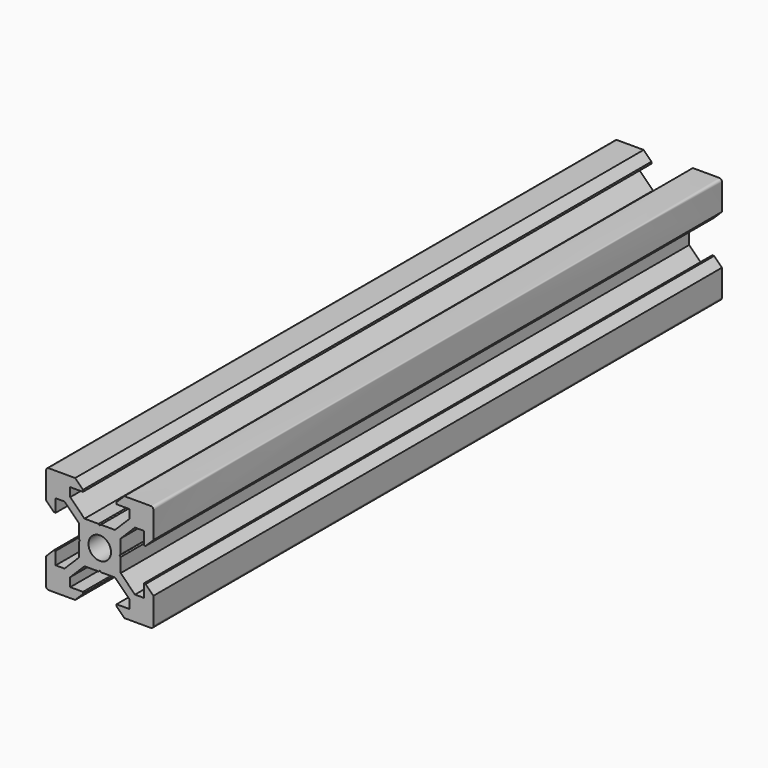
from build123d import *

# Parameters (mm, degrees)
F1_DEPTH = 132.4


# Not quite as in the source:
# - the dataset's text gives a spline's control points without its knots; the knots are read off the source's solid


with BuildPart() as f1:
    # F0 (on Front) → F1 (new body)
    with BuildSketch(Plane.XZ):
        with BuildLine():
            add(Edge.make_bspline(
                [(-8.545, 3.1250000004), (-8.43, 3.1250000004), (-8.315, 3.1250000004), (-8.2, 3.1250000004)],
                knots=[0, 0, 0, 0, 1, 1, 1, 1], degree=3))
            add(Edge.make_bspline(
                [(-8.2, 3.1250000004), (-8.2, 3.9166666671), (-8.2, 4.7083333338), (-8.2, 5.5000000004)],
                knots=[0, 0, 0, 0, 1, 1, 1, 1], degree=3))
            add(Edge.make_bspline(
                [(-8.1999999959, 5.5000000044), (-7.6535533893, 5.5000000044), (-7.1071067826, 5.5000000044), (-6.5606601759, 5.5000000044)],
                knots=[0, 0, 0, 0, 1, 1, 1, 1], degree=3))
            add(Edge.make_bspline(
                [(-6.5606601759, 5.5000000044), (-5.6737734493, 4.6131132778), (-4.7868867226, 3.7262265511), (-3.8999999959, 2.8393398244)],
                knots=[0, 0, 0, 0, 1, 1, 1, 1], degree=3))
            add(Edge.make_bspline(
                [(-3.8999999979, 2.8393398226), (-3.8999999979, 1.9628932159), (-3.8999999979, 1.0864466093), (-3.8999999979, 0.2100000026)],
                knots=[0, 0, 0, 0, 1, 1, 1, 1], degree=3))
            add(Edge.make_bspline(
                [(-3.9, 0.2100000008), (-3.83, 0.1400000008), (-3.76, 0.0700000008), (-3.69, 8e-10)],
                knots=[0, 0, 0, 0, 1, 1, 1, 1], degree=3))
            add(Edge.make_bspline(
                [(-3.9, -0.2099999992), (-3.83, -0.1399999992), (-3.76, -0.0699999992), (-3.69, 8e-10)],
                knots=[0, 0, 0, 0, 1, 1, 1, 1], degree=3))
            add(Edge.make_bspline(
                [(-3.8999999991, -2.839339821), (-3.8999999987, -1.9628932143), (-3.8999999984, -1.0864466077), (-3.899999998, -0.210000001)],
                knots=[0, 0, 0, 0, 1, 1, 1, 1], degree=3))
            add(Edge.make_bspline(
                [(-6.5606601782, -5.5000000017), (-5.6737734512, -4.6131132754), (-4.7868867241, -3.7262265491), (-3.8999999971, -2.8393398228)],
                knots=[0, 0, 0, 0, 1, 1, 1, 1], degree=3))
            add(Edge.make_bspline(
                [(-8.1999999982, -5.5000000011), (-7.6535533915, -5.5000000013), (-7.1071067849, -5.5000000015), (-6.5606601782, -5.5000000017)],
                knots=[0, 0, 0, 0, 1, 1, 1, 1], degree=3))
            add(Edge.make_bspline(
                [(-8.2000000012, -3.1249999971), (-8.2000000015, -3.9166666637), (-8.2000000019, -4.7083333304), (-8.2000000022, -5.4999999971)],
                knots=[0, 0, 0, 0, 1, 1, 1, 1], degree=3))
            add(Edge.make_bspline(
                [(-8.5450000012, -3.1249999969), (-8.4300000012, -3.124999997), (-8.3150000012, -3.124999997), (-8.2000000012, -3.1249999971)],
                knots=[0, 0, 0, 0, 1, 1, 1, 1], degree=3))
            add(Edge.make_bspline(
                [(-10.0000000018, -4.5799999963), (-9.5150000016, -4.0949999965), (-9.0300000014, -3.6099999967), (-8.5450000012, -3.1249999969)],
                knots=[0, 0, 0, 0, 1, 1, 1, 1], degree=3))
            add(Edge.make_bspline(
                [(-10.0000000038, -9.4999999963), (-10.0000000032, -7.8599999963), (-10.0000000025, -6.2199999963), (-10.0000000018, -4.5799999963)],
                knots=[0, 0, 0, 0, 1, 1, 1, 1], degree=3))
            add(Edge.make_bspline(
                [(-9.5000000039, -9.9999999965), (-9.5655199967, -9.9999999965), (-9.6293005688, -9.9873132519), (-9.6913417201, -9.9619397628), (-9.7513299005, -9.9374058943), (-9.8054004587, -9.9012771024), (-9.8535533945, -9.853553387), (-9.8995865416, -9.8079305653), (-9.9357153335, -9.7538600072), (-9.9619397702, -9.6913417126), (-9.9873132593, -9.6308520521), (-10.0000000039, -9.56707148), (-10.0000000038, -9.4999999963)],
                knots=[0, 0, 0, 0, 0.25, 0.25, 0.25, 0.5, 0.5, 0.5, 0.75, 0.75, 0.75, 1, 1, 1, 1], degree=3))
            add(Edge.make_bspline(
                [(-4.580000004, -9.9999999986), (-6.220000004, -9.9999999979), (-7.860000004, -9.9999999972), (-9.500000004, -9.9999999965)],
                knots=[0, 0, 0, 0, 1, 1, 1, 1], degree=3))
            Line((-4.580000004, -9.9999999986), (-3.1250000034, -8.5449999991))
            add(Edge.make_bspline(
                [(-3.1250000033, -8.1999999991), (-3.1250000033, -8.3149999991), (-3.1250000034, -8.4299999991), (-3.1250000034, -8.5449999991)],
                knots=[0, 0, 0, 0, 1, 1, 1, 1], degree=3))
            add(Edge.make_bspline(
                [(-5.5000000033, -8.1999999982), (-4.7083333366, -8.1999999985), (-3.91666667, -8.1999999988), (-3.1250000033, -8.1999999991)],
                knots=[0, 0, 0, 0, 1, 1, 1, 1], degree=3))
            add(Edge.make_bspline(
                [(-5.5000000066, -6.5606601742), (-5.5000000069, -7.1071067808), (-5.5000000071, -7.6535533875), (-5.5000000073, -8.1999999942)],
                knots=[0, 0, 0, 0, 1, 1, 1, 1], degree=3))
            add(Edge.make_bspline(
                [(-2.8393398255, -3.8999999953), (-3.7262265526, -4.7868867216), (-4.6131132796, -5.6737734479), (-5.5000000066, -6.5606601742)],
                knots=[0, 0, 0, 0, 1, 1, 1, 1], degree=3))
            add(Edge.make_bspline(
                [(-0.2100000015, -3.9000000003), (-1.0864466082, -3.9), (-1.9628932149, -3.8999999996), (-2.8393398215, -3.8999999993)],
                knots=[0, 0, 0, 0, 1, 1, 1, 1], degree=3))
            add(Edge.make_bspline(
                [(-1.5e-09, -3.6900000004), (-0.0700000015, -3.7600000004), (-0.1400000015, -3.8300000004), (-0.2100000015, -3.9000000003)],
                knots=[0, 0, 0, 0, 1, 1, 1, 1], degree=3))
            add(Edge.make_bspline(
                [(0.2099999985, -3.9000000005), (0.1399999985, -3.8300000005), (0.0699999985, -3.7600000005), (-1.5e-09, -3.6900000004)],
                knots=[0, 0, 0, 0, 1, 1, 1, 1], degree=3))
            add(Edge.make_bspline(
                [(2.8393398185, -3.9000000016), (1.9628932118, -3.9000000012), (1.0864466051, -3.9000000009), (0.2099999985, -3.9000000005)],
                knots=[0, 0, 0, 0, 1, 1, 1, 1], degree=3))
            add(Edge.make_bspline(
                [(5.4999999974, -6.5606601827), (4.6131132711, -5.6737734557), (3.7262265448, -4.7868867286), (2.8393398185, -3.9000000016)],
                knots=[0, 0, 0, 0, 1, 1, 1, 1], degree=3))
            add(Edge.make_bspline(
                [(5.4999999967, -8.2000000027), (5.4999999969, -7.653553396), (5.4999999971, -7.1071067894), (5.4999999974, -6.5606601827)],
                knots=[0, 0, 0, 0, 1, 1, 1, 1], degree=3))
            add(Edge.make_bspline(
                [(3.1249999967, -8.2000000017), (3.9166666634, -8.200000002), (4.70833333, -8.2000000024), (5.4999999967, -8.2000000027)],
                knots=[0, 0, 0, 0, 1, 1, 1, 1], degree=3))
            add(Edge.make_bspline(
                [(3.1249999966, -8.5450000017), (3.1249999966, -8.4300000017), (3.1249999967, -8.3150000017), (3.1249999967, -8.2000000017)],
                knots=[0, 0, 0, 0, 1, 1, 1, 1], degree=3))
            add(Edge.make_bspline(
                [(4.579999996, -10.0000000023), (4.0949999962, -9.5150000021), (3.6099999964, -9.0300000019), (3.1249999966, -8.5450000017)],
                knots=[0, 0, 0, 0, 1, 1, 1, 1], degree=3))
            add(Edge.make_bspline(
                [(9.499999996, -10.0000000043), (7.859999996, -10.0000000037), (6.219999996, -10.000000003), (4.579999996, -10.0000000023)],
                knots=[0, 0, 0, 0, 1, 1, 1, 1], degree=3))
            add(Edge.make_bspline(
                [(9.999999996, -9.5000000043), (9.999999996, -9.5655199971), (9.9873132515, -9.6293005692), (9.9619397623, -9.6913417205), (9.9374058938, -9.7513299009), (9.9012771019, -9.8054004591), (9.8535533866, -9.853553395), (9.8079305649, -9.899586542), (9.7538600068, -9.9357153339), (9.6913417122, -9.9619397706), (9.6308520517, -9.9873132598), (9.5670714797, -10.0000000043), (9.499999996, -10.0000000043)],
                knots=[0, 0, 0, 0, 0.25, 0.25, 0.25, 0.5, 0.5, 0.5, 0.75, 0.75, 0.75, 1, 1, 1, 1], degree=3))
            add(Edge.make_bspline(
                [(9.9999999981, -4.5800000043), (9.9999999974, -6.2200000043), (9.9999999967, -7.8600000043), (9.999999996, -9.5000000043)],
                knots=[0, 0, 0, 0, 1, 1, 1, 1], degree=3))
            add(Edge.make_bspline(
                [(8.5449999987, -3.1250000037), (9.0299999985, -3.6100000039), (9.5149999983, -4.0950000041), (9.9999999981, -4.5800000043)],
                knots=[0, 0, 0, 0, 1, 1, 1, 1], degree=3))
            add(Edge.make_bspline(
                [(8.1999999987, -3.1250000036), (8.3149999987, -3.1250000036), (8.4299999987, -3.1250000037), (8.5449999987, -3.1250000037)],
                knots=[0, 0, 0, 0, 1, 1, 1, 1], degree=3))
            add(Edge.make_bspline(
                [(8.1999999977, -5.5000000036), (8.199999998, -4.7083333369), (8.1999999983, -3.9166666703), (8.1999999987, -3.1250000036)],
                knots=[0, 0, 0, 0, 1, 1, 1, 1], degree=3))
            add(Edge.make_bspline(
                [(6.5606601777, -5.5000000019), (7.1071067843, -5.5000000022), (7.653553391, -5.5000000024), (8.1999999977, -5.5000000026)],
                knots=[0, 0, 0, 0, 1, 1, 1, 1], degree=3))
            add(Edge.make_bspline(
                [(3.8999999988, -2.8393398208), (4.7868867251, -3.7262265479), (5.6737734514, -4.6131132749), (6.5606601777, -5.5000000019)],
                knots=[0, 0, 0, 0, 1, 1, 1, 1], degree=3))
            add(Edge.make_bspline(
                [(3.8999999999, -0.2100000008), (3.8999999995, -1.0864466075), (3.8999999991, -1.9628932142), (3.8999999988, -2.8393398208)],
                knots=[0, 0, 0, 0, 1, 1, 1, 1], degree=3))
            add(Edge.make_bspline(
                [(3.69, -8e-10), (3.76, -0.0700000008), (3.8299999999, -0.1400000008), (3.8999999999, -0.2100000008)],
                knots=[0, 0, 0, 0, 1, 1, 1, 1], degree=3))
            add(Edge.make_bspline(
                [(3.69, -8e-10), (3.76, 0.0699999992), (3.83, 0.1399999992), (3.9, 0.2099999992)],
                knots=[0, 0, 0, 0, 1, 1, 1, 1], degree=3))
            add(Edge.make_bspline(
                [(3.9, 0.2099999992), (3.9, 1.0864466059), (3.9, 1.9628932126), (3.9, 2.8393398192)],
                knots=[0, 0, 0, 0, 1, 1, 1, 1], degree=3))
            add(Edge.make_bspline(
                [(3.9, 2.8393398192), (4.7868867266, 3.7262265459), (5.6737734533, 4.6131132726), (6.5606601799, 5.4999999992)],
                knots=[0, 0, 0, 0, 1, 1, 1, 1], degree=3))
            add(Edge.make_bspline(
                [(6.5606601799, 5.4999999992), (7.1071067866, 5.4999999992), (7.6535533933, 5.4999999992), (8.2, 5.4999999992)],
                knots=[0, 0, 0, 0, 1, 1, 1, 1], degree=3))
            add(Edge.make_bspline(
                [(8.2, 5.5000000002), (8.2, 4.7083333336), (8.2, 3.9166666669), (8.2, 3.1250000002)],
                knots=[0, 0, 0, 0, 1, 1, 1, 1], degree=3))
            add(Edge.make_bspline(
                [(8.2, 3.1250000002), (8.315, 3.1250000002), (8.43, 3.1250000002), (8.545, 3.1250000002)],
                knots=[0, 0, 0, 0, 1, 1, 1, 1], degree=3))
            add(Edge.make_bspline(
                [(8.545, 3.1250000002), (9.03, 3.6100000002), (9.515, 4.0950000002), (10, 4.5800000002)],
                knots=[0, 0, 0, 0, 1, 1, 1, 1], degree=3))
            add(Edge.make_bspline(
                [(10, 4.5800000002), (10, 6.2200000002), (10, 7.8600000002), (10, 9.5000000002)],
                knots=[0, 0, 0, 0, 1, 1, 1, 1], degree=3))
            add(Edge.make_bspline(
                [(10, 9.5000000002), (10, 9.565519993), (9.9873132554, 9.6293005651), (9.9619397663, 9.6913417164), (9.9374058978, 9.7513298969), (9.901277106, 9.805400455), (9.8535533907, 9.8535533909), (9.807930569, 9.899586538), (9.7538600108, 9.9357153299), (9.6913417163, 9.9619397666), (9.6308520558, 9.9873132558), (9.5670714838, 10.0000000004), (9.5, 10.0000000004)],
                knots=[0, 0, 0, 0, 0.25, 0.25, 0.25, 0.5, 0.5, 0.5, 0.75, 0.75, 0.75, 1, 1, 1, 1], degree=3))
            add(Edge.make_bspline(
                [(9.5, 10.0000000004), (7.86, 10.0000000004), (6.22, 10.0000000004), (4.58, 10.0000000004)],
                knots=[0, 0, 0, 0, 1, 1, 1, 1], degree=3))
            add(Edge.make_bspline(
                [(4.58, 10.0000000004), (4.095, 9.5150000004), (3.61, 9.0300000004), (3.125, 8.5450000004)],
                knots=[0, 0, 0, 0, 1, 1, 1, 1], degree=3))
            add(Edge.make_bspline(
                [(3.125, 8.5450000004), (3.125, 8.4300000004), (3.125, 8.3150000004), (3.125, 8.2000000004)],
                knots=[0, 0, 0, 0, 1, 1, 1, 1], degree=3))
            add(Edge.make_bspline(
                [(3.125, 8.2000000004), (3.9166666667, 8.2000000004), (4.7083333334, 8.2000000004), (5.5, 8.2000000004)],
                knots=[0, 0, 0, 0, 1, 1, 1, 1], degree=3))
            add(Edge.make_bspline(
                [(5.5, 8.2000000004), (5.5, 7.6535533938), (5.5, 7.1071067871), (5.5, 6.5606601804)],
                knots=[0, 0, 0, 0, 1, 1, 1, 1], degree=3))
            add(Edge.make_bspline(
                [(5.5, 6.5606601804), (4.6131132734, 5.6737734538), (3.7262265467, 4.7868867271), (2.8393398201, 3.9000000004)],
                knots=[0, 0, 0, 0, 1, 1, 1, 1], degree=3))
            add(Edge.make_bspline(
                [(2.8393398201, 3.9000000004), (1.9628932134, 3.9000000004), (1.0864466067, 3.9000000004), (0.21, 3.9000000004)],
                knots=[0, 0, 0, 0, 1, 1, 1, 1], degree=3))
            add(Edge.make_bspline(
                [(0.21, 3.9000000004), (0.14, 3.8300000004), (0.07, 3.7600000004), (0, 3.6900000004)],
                knots=[0, 0, 0, 0, 1, 1, 1, 1], degree=3))
            add(Edge.make_bspline(
                [(0, 3.6900000004), (-0.07, 3.7600000004), (-0.14, 3.8300000004), (-0.21, 3.9000000004)],
                knots=[0, 0, 0, 0, 1, 1, 1, 1], degree=3))
            add(Edge.make_bspline(
                [(-0.21, 3.9000000004), (-1.0864466066, 3.9000000004), (-1.9628932133, 3.9000000004), (-2.8393398199, 3.9000000004)],
                knots=[0, 0, 0, 0, 1, 1, 1, 1], degree=3))
            add(Edge.make_bspline(
                [(-2.8393398239, 3.8999999964), (-3.7262265506, 4.7868867231), (-4.6131132773, 5.6737734498), (-5.5000000039, 6.5606601764)],
                knots=[0, 0, 0, 0, 1, 1, 1, 1], degree=3))
            add(Edge.make_bspline(
                [(-5.5, 6.5606601804), (-5.5, 7.1071067871), (-5.5, 7.6535533938), (-5.5, 8.2000000004)],
                knots=[0, 0, 0, 0, 1, 1, 1, 1], degree=3))
            add(Edge.make_bspline(
                [(-5.5, 8.2000000004), (-4.7083333333, 8.2000000004), (-3.9166666666, 8.2000000004), (-3.125, 8.2000000004)],
                knots=[0, 0, 0, 0, 1, 1, 1, 1], degree=3))
            add(Edge.make_bspline(
                [(-3.125, 8.2000000004), (-3.125, 8.3150000004), (-3.125, 8.4300000004), (-3.125, 8.5450000004)],
                knots=[0, 0, 0, 0, 1, 1, 1, 1], degree=3))
            Line((-3.125, 8.5450000004), (-4.58, 10.0000000004))
            add(Edge.make_bspline(
                [(-4.58, 10.0000000004), (-6.22, 10.0000000004), (-7.86, 10.0000000004), (-9.5, 10.0000000004)],
                knots=[0, 0, 0, 0, 1, 1, 1, 1], degree=3))
            add(Edge.make_bspline(
                [(-9.4999999998, 10.0000000004), (-9.5655199926, 10.0000000005), (-9.6293005647, 9.9873132559), (-9.691341716, 9.9619397667), (-9.7513298965, 9.9374058983), (-9.8054004546, 9.9012771064), (-9.8535533905, 9.8535533911), (-9.8995865376, 9.8079305694), (-9.9357153295, 9.7538600112), (-9.9619397662, 9.6913417167), (-9.9873132554, 9.6308520562), (-10, 9.5670714842), (-10, 9.5000000004)],
                knots=[0, 0, 0, 0, 0.25, 0.25, 0.25, 0.5, 0.5, 0.5, 0.75, 0.75, 0.75, 1, 1, 1, 1], degree=3))
            add(Edge.make_bspline(
                [(-10, 9.5000000004), (-10, 7.8600000004), (-10, 6.2200000004), (-10, 4.5800000004)],
                knots=[0, 0, 0, 0, 1, 1, 1, 1], degree=3))
            add(Edge.make_bspline(
                [(-10, 4.5800000004), (-9.515, 4.0950000004), (-9.03, 3.6100000004), (-8.545, 3.1250000004)],
                knots=[0, 0, 0, 0, 1, 1, 1, 1], degree=3))
        make_face()
        with BuildLine():
            add(Edge.make_bspline(
                [(2.1, -4e-10), (2.1000000002, 0.2748893568), (1.9906569307, 0.8245399239), (1.5235828541, 1.5235874774), (0.8245570992, 1.9906556095), (5e-10, 2.1546721958), (-0.8245570982, 1.9906556098), (-1.5235828533, 1.523587478), (-1.9906569302, 0.8245399247), (-2.1, 0.2748893577), (-2.1, 4e-10)],
                knots=[-3.1415926536, -3.1415926536, -3.1415926536, -3.1415926536, -2.7488935719, -2.3561944902, -1.9634954085, -1.5707963268, -1.1780972451, -0.7853981634, -0.3926990817, 0, 0, 0, 0], degree=3))
            add(Edge.make_bspline(
                [(2.1, -4e-10), (2.1, -0.2748893577), (1.9906569304, -0.8245399247), (1.5235828534, -1.523587478), (0.8245570983, -1.9906556098), (-4e-10, -2.1546721958), (-0.824557099, -1.9906556095), (-1.5235828539, -1.5235874774), (-1.9906569306, -0.8245399239), (-2.1, -0.2748893568), (-2.1, 4e-10)],
                knots=[-3.1415926536, -3.1415926536, -3.1415926536, -3.1415926536, -2.7488935719, -2.3561944902, -1.9634954085, -1.5707963268, -1.1780972451, -0.7853981634, -0.3926990817, 0, 0, 0, 0], degree=3))
        make_face(mode=Mode.SUBTRACT)
    extrude(amount=-F1_DEPTH)


solid = f1.part
